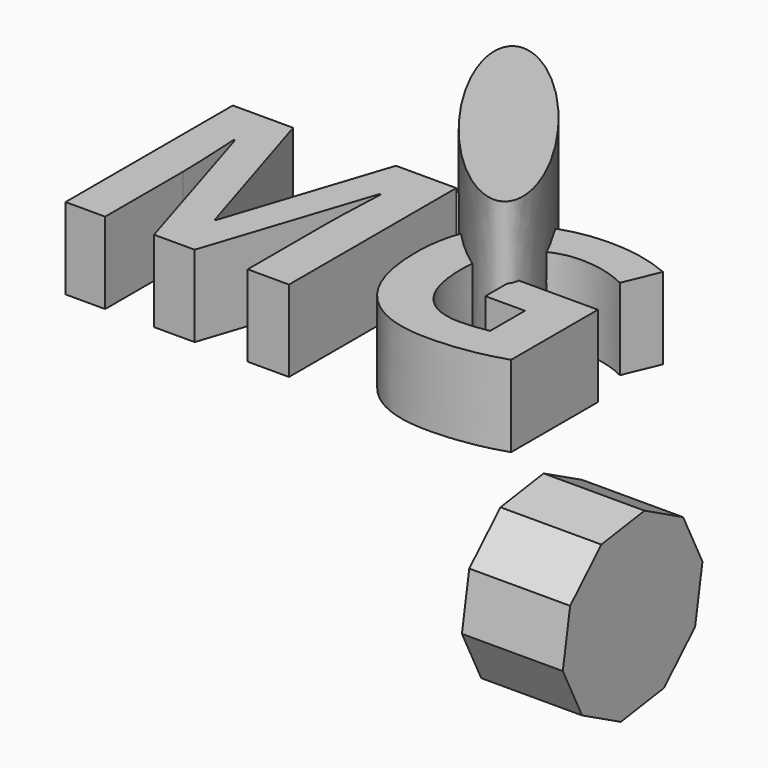
from build123d import *

# Parameters (mm, degrees)
F1_DEPTH     = 48.006
F2_TEXT_SIZE = 91.4164353162
F3_DEPTH     = 25.4
F5_DEPTH     = 31.496


# Not quite as in the source:
# - Text() gives the source's letters only with a copy of the font that has no kerning and outlines rounded to 1/6400 em; it was checked with that copy


with BuildPart() as f1:
    # F0 (on Top) → F1 (new body)
    with BuildSketch(Plane.XY):
        with BuildLine():
            add(Edge.make_bspline(
                [(-35.7876941562, -32.6467752457), (-19.0310146919, -19.893806531), (-64.6789671983, 22.6998719802), (-110.3269197047, 65.2935504913), (-81.4356466625, 9.9469032655), (-52.5443736204, -45.3997439603), (-35.7876941562, -32.6467752457)],
                knots=[0, 0, 0, 2.0943951024, 2.0943951024, 4.1887902048, 4.1887902048, 6.2831853072, 6.2831853072, 6.2831853072], degree=2, weights=[1, 0.5, 1, 0.5, 1, 0.5, 1]))
        make_face()
    extrude(amount=F1_DEPTH)


with BuildPart() as f3:
    # F2 (on Top) → F3 (new body)
    with BuildSketch(Plane.XY):
        with Locations((-154.5137717241, -65.8198334277)):
            Text('MG', F2_TEXT_SIZE, font='Open Sans', font_style=FontStyle.BOLD, text_align=(TextAlign.LEFT, TextAlign.BOTTOM))
    extrude(amount=F3_DEPTH)


with BuildPart() as f5:
    # F4 (on Right) → F5 (new body)
    with BuildSketch(Plane.YZ):
        Polygon((-47.067392489, -11.0096876603), (-62.1385240349, -3.1024579796), (-78.9790785728, -5.5639636475), (-91.1565366587, -17.4539931624), (-94.0195232002, -34.2309593769), (-86.4744746479, -49.486631425), (-71.403343102, -57.3938611057), (-54.5627885641, -54.9323554378), (-42.3853304783, -43.0423259229), (-39.5223439367, -26.2653597085), align=None)
    extrude(amount=F5_DEPTH)


solid = Compound([f1.part, f3.part, f5.part])
